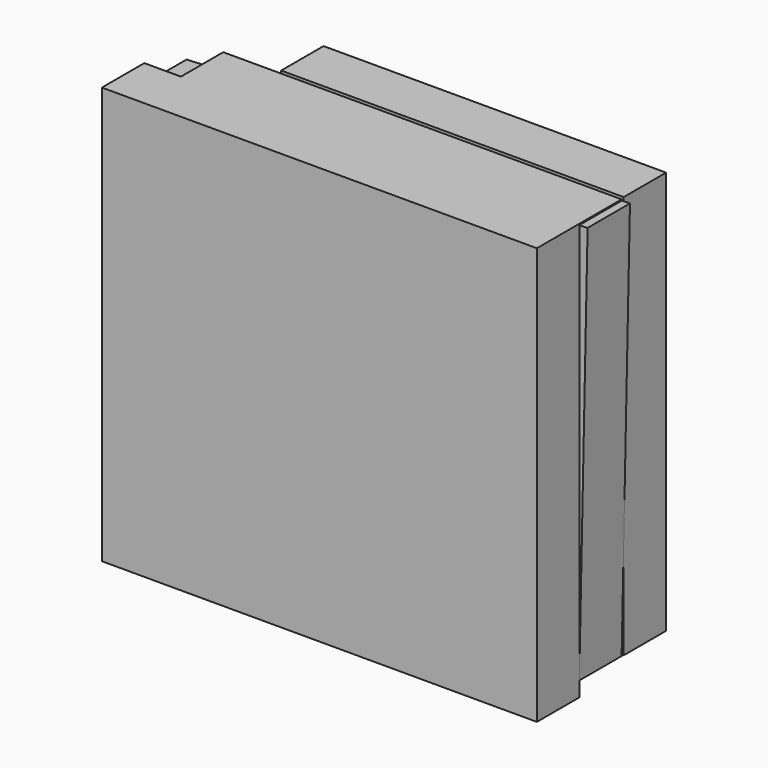
from build123d import *

# Parameters (mm, degrees)
F0_W      = 191.0914182663
F0_H      = 192.8930431604
F1_DEPTH  = 25.4
F2_W      = 25.4
F2_H      = 25.5114277713
F3_DEPTH  = 25.4
F4_W      = 125.7558986545
F4_H      = 7.1474313736
F4_H_2    = 192.8930431604
F4_W_2    = 50.9491413832
F5_DEPTH  = 25.4
F7_DEPTH  = 25.4
F9_W      = 164.3103808165
F9_H      = 10.6280595064
F10_DEPTH = 25.4


with BuildPart() as f1:
    # F0 (on Front) → F1 (new body)
    with BuildSketch(Plane.XZ):
        with Locations((-0.6164610386, -0.6837919354)):
            Rectangle(F0_W, F0_H)
        Polygon((0, 75.5859687924), (74.6201202273, 75.5859687924), (74.6201202273, 11.123508215), (81.607028842, -13.4125072509), (74.6201202273, -13.2084926445), (74.6201202273, -76.0672464967), (0, -76.0672464967), (-77.7053460479, -76.0672464967), (-77.7053460479, -8.7606571615), (-77.7053460479, 12.5154424459), (-77.7053460479, 75.5859687924), align=None, mode=Mode.SUBTRACT)
    extrude(amount=F1_DEPTH)

    # F2 (on face) → F3 (join)
    with BuildSketch(Plane(origin=(71.9530620256, 0, 20.4894502783), x_dir=(0, -1, 0), z_dir=(-0.9617656717, 0, -0.2738736803))):
        with Locations((12.7, -22.4939924905)):
            Rectangle(F2_W, F2_H)
    extrude(amount=F3_DEPTH)

    # F4 (on face) → F5 (join)
    with BuildSketch(Plane.XZ.offset(25.4)):
        with Locations((32.0512987673, -100.7040292025)):
            Rectangle(F4_W, F4_H)
        with Locations((32.0512987673, -0.6837919354)):
            Rectangle(F4_W, F4_H_2)
        Polygon((-30.8266505599, -104.2777448893), (-30.8266505599, -97.1303135157), (-81.7757919431, -97.1303135157), (-81.7757919431, 95.7627296448), (-113.723911345, 95.7627296448), (-113.723911345, -104.2777448893), align=None)
        with Locations((-56.3012212515, -0.6837919354)):
            Rectangle(F4_W_2, F4_H_2)
    extrude(amount=F5_DEPTH)

    # F6 (on face) → F7 (join)
    with BuildSketch(Plane(origin=(0, -25.4, 0), x_dir=(-1, 0, 0), z_dir=(0, 1, 0))):
        Polygon((-98.9333018661, 95.3389704227), (-94.9292480946, -97.1303135157), (113.723911345, -97.1303135157), (113.723911345, 86.9726911187), align=None)
    extrude(amount=F7_DEPTH)

    # F9 (on face) → F10 (join)
    with BuildSketch(Plane(origin=(0, 0, 0), x_dir=(-1, 0, 0), z_dir=(0, 1, 0))):
        Polygon((-95.9361866117, 86.4189863205), (-95.9361866117, -96.4786112309), (73.3251571655, -96.4786112309), (73.3251571655, 86.4189863205), (68.3741942048, 86.4189863205), align=None)
        with Locations((-13.7809962034, 91.7330160737)):
            Rectangle(F9_W, F9_H)
    extrude(amount=F10_DEPTH)


solid = f1.part
